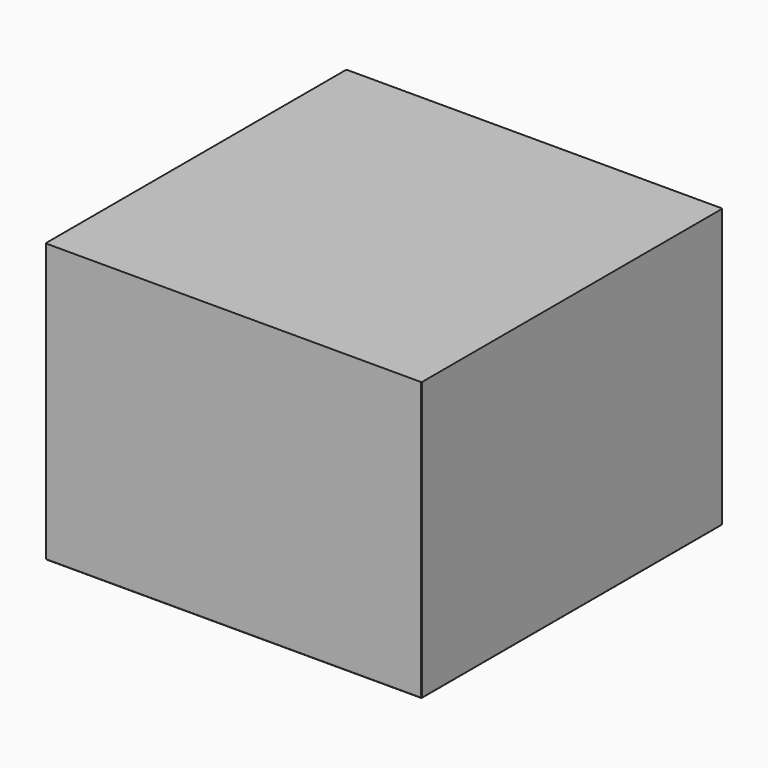
from build123d import *

# Parameters (mm, degrees)
F0_W     = 270
F0_H     = 200
F1_DEPTH = 270
F2_SIZE  = 0.5


with BuildPart() as f1:
    # F0 (on Front) → F1 (new body)
    with BuildSketch(Plane.XZ):
        with Locations((-135, 100)):
            Rectangle(F0_W, F0_H)
    extrude(amount=-F1_DEPTH)

    # F2
    f2_edges = [f1.edges().sort_by_distance(p)[0] for p in [
        (0, 0, 100),
        (0, 270, 100),
        (-270, 0, 100),
        (-270, 270, 100),
        (-270, 135, 0),
        (0, 135, 0),
        (-135, 0, 0),
        (-135, 270, 0),
    ]]
    chamfer(f2_edges, length=F2_SIZE)


solid = f1.part
